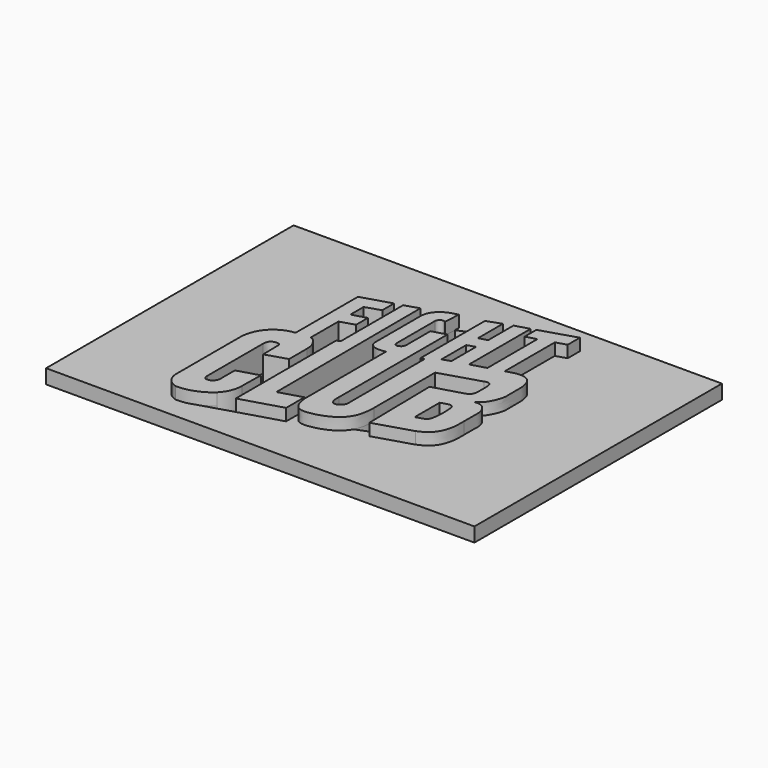
from build123d import *

# Parameters (mm, degrees)
F0_W     = 90
F0_H     = 65
F1_DEPTH = 3
F2_DEPTH = 5.5
F4_DEPTH = 25


# Not quite as in the source:
# - a feature names something its author has since deleted; it is built from what else it names


with BuildPart() as f1:
    # F0 (on Top) → F1 (new body)
    with BuildSketch(Plane.XY):
        Rectangle(F0_W, F0_H)
        with BuildLine():
            Line((-11.7899651246, 17.3868578509), (-11.7899651246, 14.2935177732))
            Line((-11.7899651246, 14.2935177732), (-14.9118620558, 13.28190385))
            Line((-14.9118620558, 13.28190385), (-14.9118620558, 9.8245825553))
            Line((-14.9118620558, 9.8245825553), (-14.8359441439, 9.8464276794))
            Line((-14.8359441439, 9.8464276794), (-11.9289977815, 10.6828917294))
            Line((-11.9289977815, 10.6828917294), (-11.9289977815, 7.5737699435))
            Line((-11.9289977815, 7.5737699435), (-14.9118620558, 6.6583940559))
            Line((-14.9118620558, 6.6583940559), (-14.9118620558, -0.6190531353))
            Line((-14.9118620558, -0.6190531353), (-14.8359441439, -0.6190531353))
            add(Edge.make_bspline(
                [(-12.8983538912, -4.1546191569), (-12.9124355164, -3.4646401315), (-13.0426874661, -2.4052822087), (-14.1635179222, -0.8313651281), (-14.6513370426, -0.6795562339), (-14.8359441439, -0.6190531353)],
                knots=[0, 0, 0, 0, 0.3871210779, 0.7691695686, 1, 1, 1, 1], degree=3))
            Line((-12.8983538912, -4.1546191569), (-12.8983538912, -8.8000393834))
            Line((-12.8983538912, -8.8000393834), (-17.270977576, -10.1718452605))
            Line((-17.270977576, -10.1718452605), (-17.3239837629, -6.5835107489))
            add(Edge.make_bspline(
                [(-19.649932717, -7.1929238033), (-19.6340625481, -6.6727895144), (-19.4415656957, -6.0485860746), (-18.7104823295, -5.5186813522), (-17.3236080712, -5.4227422638), (-17.3243871941, -6.203783376), (-17.3239837629, -6.5835107489)],
                knots=[0, 0, 0, 0, 0.266822824, 0.4960878337, 0.7560668313, 1, 1, 1, 1], degree=3))
            Line((-19.649932717, -7.1929238033), (-19.649932717, -21.7389181386))
            add(Edge.make_bspline(
                [(-18.3777159405, -22.8102611267), (-18.7096900591, -22.8762786233), (-19.33843798, -23.0013135624), (-19.6405821898, -22.1927150073), (-19.6470449505, -21.8790663219), (-19.649932717, -21.7389181386)],
                knots=[0, 0, 0, 0, 0.3822506469, 0.7239699906, 1, 1, 1, 1], degree=3))
            ThreePointArc((-18.3777159405, -22.8102611267), (-17.6136064221, -22.2363913544), (-17.3231101454, -21.3260058399))
            Line((-17.3231101454, -21.3260058399), (-17.3231101454, -17.5101269313))
            Line((-17.3231101454, -17.5101269313), (-12.8908924283, -16.2136158955))
            Line((-12.8908924283, -16.2136158955), (-12.9712542512, -21.1030652423))
            ThreePointArc((-12.9712542512, -21.1030652423), (-13.4353650173, -23.4585093269), (-14.7708491992, -25.4535024695))
            ThreePointArc((-14.7708491992, -25.4535024695), (-17.8496394574, -27.3225084243), (-21.3954732545, -27.9543275408))
            ThreePointArc((-21.3954732545, -27.9543275408), (-23.3162452582, -26.6851378839), (-24.0600023068, -24.5063692115))
            Line((-24.0600023068, -24.5063692115), (-24.0600023068, -8.0969591465))
            ThreePointArc((-24.0600023068, -8.0969591465), (-23.8409881388, -6.008395119), (-23.0513839577, -4.0624783325))
            ThreePointArc((-23.0513839577, -4.0624783325), (-20.856584496, -1.8407427995), (-17.897732893, -0.8415177762))
            Line((-17.897732893, -0.8415177762), (-17.897732893, 15.5245404617))
            Line((-17.897732893, 15.5245404617), (-11.7899651246, 17.3868578509))
        make_face(mode=Mode.SUBTRACT)
        Polygon((-10.2390258983, 17.8220402536), (-7.3459431316, 18.7296739119), (-7.2041264371, -19.249136779), (-2.439048632, -17.8309577456), (-2.439048632, -22.6527638219), (-10.9764799627, -25.2054852029), (-10.9764799627, 1.1442654634), (-10.2390258983, 1.3995376015), align=None, mode=Mode.SUBTRACT)
        with BuildLine():
            add(Edge.make_bspline(
                [(-1.0214279034, 20.9294296394), (-1.795044013, 20.7272698748), (-3.3218007923, 20.3406175558), (-5.1422433593, 18.8024410524), (-5.5532558817, 17.434179196), (-5.6010190581, 16.6460884355)],
                knots=[0, 0, 0, 0, 0.3420427267, 0.6738343467, 1, 1, 1, 1], degree=3))
            Line((-1.0214279034, 20.9294296394), (-1.1788295361, 17.5223806532))
            ThreePointArc((-1.1788295361, 17.5223806532), (-1.3659565648, 17.6186204532), (-1.5723679927, 17.6595221205))
            ThreePointArc((-1.5723679927, 17.6595221205), (-2.3268435709, 17.3860281515), (-2.645024017, 16.6492829086))
            Line((-2.645024017, 16.6492829086), (-2.645024017, 6.6834372087))
            add(Edge.make_bspline(
                [(-0.975842239, 7.3917701397), (-0.9782823928, 7.3091479001), (-0.9566797659, 7.1256039043), (-1.0681286366, 6.5441772072), (-1.3929022467, 6.1116799848), (-2.5109116823, 5.7508045045), (-2.6580041052, 6.412182815), (-2.645024017, 6.6834372087)],
                knots=[0, 0, 0, 0, 0.1336018541, 0.3279707081, 0.5240102199, 0.7751644105, 1, 1, 1, 1], degree=3))
            Line((-0.975842239, 7.3917701397), (-0.975842239, 13.4126014265))
            Line((-0.975842239, 13.4126014265), (1.9419226264, 14.2566961684))
            Line((1.9419226264, 14.2566961684), (1.9419226264, -14.2681037451))
            add(Edge.make_bspline(
                [(4.4582015212, -14.2681037451), (4.4582015212, -14.4613851485), (4.6185530783, -15.2735437801), (3.810378959, -16.3402712665), (2.669439425, -16.7790884746), (1.8680807242, -15.7743077401), (1.9702860752, -14.8211937439), (1.9419226264, -14.2681037451)],
                knots=[0, 0, 0, 0, 0.1782994827, 0.39186138, 0.5816412367, 0.7692567527, 1, 1, 1, 1], degree=3))
            Line((4.4582015212, -14.2681037451), (4.4582015212, 5.1330709979))
            Line((4.4582015212, 5.1330709979), (3.7308113658, 4.9677546006))
            Line((3.7308113658, 4.9677546006), (3.7308113658, 21.8574482525))
            Line((3.7308113658, 21.8574482525), (6.6653340971, 22.8784648276))
            Line((6.6653340971, 22.8784648276), (6.6653340971, 16.368545091))
            Line((6.6653340971, 16.368545091), (8.419302035, 16.8407677776))
            Line((8.419302035, 16.8407677776), (8.419302035, 23.4856081248))
            Line((8.419302035, 23.4856081248), (11.3538244915, 24.3288611169))
            Line((11.3538244915, 24.3288611169), (11.3538244915, 8.1383883934))
            Line((11.3538244915, 8.1383883934), (14.4907289629, 9.0491027897))
            Line((14.4907289629, 9.0491027897), (14.4907289629, 22.1701313472))
            Line((14.4907289629, 22.1701313472), (12.2982687658, 21.56298805))
            Line((12.2982687658, 21.56298805), (12.2982687658, 24.6324316666))
            Line((12.2982687658, 24.6324316666), (19.6177110671, 26.9260831458))
            Line((19.6177110671, 26.9260831458), (19.6177110671, 23.7217178197))
            Line((19.6177110671, 23.7217178197), (17.4389254567, 23.0471158656))
            Line((17.4389254567, 23.0471158656), (17.4389254567, 9.9340454692))
            Line((17.4389254567, 9.9340454692), (17.5568187673, 9.9340454692))
            add(Edge.make_bspline(
                [(23.3318888071, -8.1512481567), (23.3311911227, -7.4858005871), (23.3307677799, -6.4709077438), (23.3343646105, -5.0115116682), (23.3288725027, -4.9910573322), (23.4432301916, -3.9602161044), (22.7653981413, -2.4247467881), (21.4983184593, -1.5549434987), (19.998240636, -1.8718939633), (21.2623812155, -1.1033143641), (22.0502922664, -0.3456082574), (23.2245036891, 2.2173413762), (23.1970215174, 3.8249680988), (23.1643405632, 6.7270889592), (23.1681424876, 7.3536889688), (22.7894330471, 9.4422107912), (21.4631720563, 10.4647739779), (19.6042894167, 10.627637088), (18.2733323534, 10.1767682526), (17.5568187673, 9.9340454692)],
                knots=[0, 0, 0, 0, 0.0686633322, 0.1241792585, 0.1317609375, 0.1781168183, 0.2439866183, 0.3061193494, 0.3529473951, 0.3988783877, 0.455494654, 0.5360218639, 0.6036835088, 0.6857463768, 0.7281580678, 0.797518151, 0.8604110332, 0.9264215245, 1, 1, 1, 1], degree=3))
            add(Edge.make_bspline(
                [(19.2568509865, -15.8505986956), (19.5510345612, -15.7266917741), (20.2459241451, -15.4339755), (21.9033973633, -14.3394960858), (22.9170105079, -12.421003478), (23.3512677684, -10.475815106), (23.3305495269, -8.9474042322), (23.3318888071, -8.1512481567)],
                knots=[0, 0, 0, 0, 0.1499469204, 0.3543171151, 0.5693051427, 0.7758772125, 1, 1, 1, 1], degree=3))
            Line((19.2568509865, -15.8505986956), (11.5152085686, -18.23727121))
            Line((11.5152085686, -18.23727121), (11.2434201144, -2.1050125944))
            Line((11.2434201144, -2.1050125944), (17.0577787685, -0.4173805913))
            add(Edge.make_bspline(
                [(17.0577787685, 4.9326692384), (17.2359444971, 5.0062828452), (17.5963985204, 5.1552133997), (18.3004216541, 5.0379598376), (18.5868743443, 4.0594275645), (18.5659774666, 3.2509662277), (18.6012430245, 1.112721129), (18.3101521273, 0.2135182891), (17.6915830324, -0.2066600599), (17.2685862853, -0.34729354), (17.0577787685, -0.4173805913)],
                knots=[0, 0, 0, 0, 0.1016144921, 0.2055802359, 0.3310055102, 0.4574330561, 0.651788574, 0.7805878019, 0.8906522546, 1, 1, 1, 1], degree=3))
            Line((17.0577787685, 4.9326692384), (8.8136700145, 2.4044824988))
            Line((8.8136700145, 2.4044824988), (8.8136700145, -13.70638746))
            add(Edge.make_bspline(
                [(-2.1296884432, -18.019118476), (-2.0995822923, -18.6635207362), (-1.857078119, -19.823460143), (-1.4816179926, -20.7110735924), (-0.7399237684, -21.5449777161), (0.5509044259, -21.8812292133), (3.1831892549, -21.4471075773), (6.0217835741, -20.2553038527), (7.6687373415, -18.601967223), (8.4960625988, -16.8878330756), (8.8140079, -14.7485973532), (8.8137678216, -14.0086200559), (8.8136700145, -13.70638746)],
                knots=[0, 0, 0, 0, 0.1027277517, 0.1769473417, 0.2532577584, 0.3376408889, 0.4609102569, 0.5950787177, 0.7085765562, 0.813280218, 0.9237370973, 1, 1, 1, 1], degree=3))
            Line((-2.1296884432, -18.019118476), (-2.1296884432, 3.1618176804))
            Line((-2.1296884432, 3.1618176804), (-2.2223336581, 3.1618176804))
            add(Edge.make_bspline(
                [(-5.6010190581, 4.5141229309), (-5.5493043432, 3.954976001), (-4.844515491, 3.1292890206), (-3.2977966838, 2.9514441965), (-2.5561304606, 3.0983845963), (-2.2223336581, 3.1618176804)],
                knots=[0, 0, 0, 0, 0.3499782987, 0.7004813403, 1, 1, 1, 1], degree=3))
            Line((-5.6010190581, 4.5141229309), (-5.6010190581, 16.6460884355))
        make_face(mode=Mode.SUBTRACT)
    extrude(amount=F1_DEPTH)

    # F0 (on Top) → F2 (join)
    with BuildSketch(Plane.XY):
        with BuildLine():
            Line((-14.9118620558, 13.28190385), (-11.7899651246, 14.2935177732))
            Line((-11.7899651246, 14.2935177732), (-11.7899651246, 17.3868578509))
            Line((-11.7899651246, 17.3868578509), (-17.897732893, 15.5245404617))
            Line((-17.897732893, 15.5245404617), (-17.897732893, -0.8415177762))
            ThreePointArc((-17.897732893, -0.8415177762), (-20.856584496, -1.8407427995), (-23.0513839577, -4.0624783325))
            ThreePointArc((-23.0513839577, -4.0624783325), (-23.8409881388, -6.008395119), (-24.0600023068, -8.0969591465))
            Line((-24.0600023068, -8.0969591465), (-24.0600023068, -24.5063692115))
            ThreePointArc((-24.0600023068, -24.5063692115), (-23.3162452582, -26.6851378839), (-21.3954732545, -27.9543275408))
            ThreePointArc((-21.3954732545, -27.9543275408), (-17.8496394574, -27.3225084243), (-14.7708491992, -25.4535024695))
            ThreePointArc((-14.7708491992, -25.4535024695), (-13.4353650173, -23.4585093269), (-12.9712542512, -21.1030652423))
            Line((-12.9712542512, -21.1030652423), (-12.8908924283, -16.2136158955))
            Line((-12.8908924283, -16.2136158955), (-17.3231101454, -17.5101269313))
            Line((-17.3231101454, -17.5101269313), (-17.3231101454, -21.3260058399))
            ThreePointArc((-17.3231101454, -21.3260058399), (-17.6136064221, -22.2363913544), (-18.3777159405, -22.8102611267))
            add(Edge.make_bspline(
                [(-18.3777159405, -22.8102611267), (-18.7096900591, -22.8762786233), (-19.33843798, -23.0013135624), (-19.6405821898, -22.1927150073), (-19.6470449505, -21.8790663219), (-19.649932717, -21.7389181386)],
                knots=[0, 0, 0, 0, 0.3822506469, 0.7239699906, 1, 1, 1, 1], degree=3))
            Line((-19.649932717, -21.7389181386), (-19.649932717, -7.1929238033))
            add(Edge.make_bspline(
                [(-19.649932717, -7.1929238033), (-19.6340625481, -6.6727895144), (-19.4415656957, -6.0485860746), (-18.7104823295, -5.5186813522), (-17.3236080712, -5.4227422638), (-17.3243871941, -6.203783376), (-17.3239837629, -6.5835107489)],
                knots=[0, 0, 0, 0, 0.266822824, 0.4960878337, 0.7560668313, 1, 1, 1, 1], degree=3))
            Line((-17.3239837629, -6.5835107489), (-17.270977576, -10.1718452605))
            Line((-17.270977576, -10.1718452605), (-12.8983538912, -8.8000393834))
            Line((-12.8983538912, -8.8000393834), (-12.8983538912, -4.1546191569))
            add(Edge.make_bspline(
                [(-12.8983538912, -4.1546191569), (-12.9124355164, -3.4646401315), (-13.0426874661, -2.4052822087), (-14.1635179222, -0.8313651281), (-14.6513370426, -0.6795562339), (-14.8359441439, -0.6190531353)],
                knots=[0, 0, 0, 0, 0.3871210779, 0.7691695686, 1, 1, 1, 1], degree=3))
            Line((-14.8359441439, -0.6190531353), (-14.9118620558, -0.6190531353))
            Line((-14.9118620558, -0.6190531353), (-14.9118620558, 6.6583940559))
            Line((-14.9118620558, 6.6583940559), (-11.9289977815, 7.5737699435))
            Line((-11.9289977815, 7.5737699435), (-11.9289977815, 10.6828917294))
            Line((-11.9289977815, 10.6828917294), (-14.8359441439, 9.8464276794))
            Line((-14.8359441439, 9.8464276794), (-14.9118620558, 9.8245825553))
            Line((-14.9118620558, 9.8245825553), (-14.9118620558, 13.28190385))
        make_face()
        Polygon((-7.2041264371, -19.249136779), (-7.3459431316, 18.7296739119), (-10.2390258983, 17.8220402536), (-10.2390258983, 1.3995376015), (-10.9764799627, 1.1442654634), (-10.9764799627, -25.2054852029), (-2.439048632, -22.6527638219), (-2.439048632, -17.8309577456), align=None)
        with BuildLine():
            Line((-1.1788295361, 17.5223806532), (-1.0214279034, 20.9294296394))
            add(Edge.make_bspline(
                [(-1.0214279034, 20.9294296394), (-1.795044013, 20.7272698748), (-3.3218007923, 20.3406175558), (-5.1422433593, 18.8024410524), (-5.5532558817, 17.434179196), (-5.6010190581, 16.6460884355)],
                knots=[0, 0, 0, 0, 0.3420427267, 0.6738343467, 1, 1, 1, 1], degree=3))
            Line((-5.6010190581, 16.6460884355), (-5.6010190581, 4.5141229309))
            add(Edge.make_bspline(
                [(-5.6010190581, 4.5141229309), (-5.5493043432, 3.954976001), (-4.844515491, 3.1292890206), (-3.2977966838, 2.9514441965), (-2.5561304606, 3.0983845963), (-2.2223336581, 3.1618176804)],
                knots=[0, 0, 0, 0, 0.3499782987, 0.7004813403, 1, 1, 1, 1], degree=3))
            Line((-2.2223336581, 3.1618176804), (-2.1296884432, 3.1618176804))
            Line((-2.1296884432, 3.1618176804), (-2.1296884432, -18.019118476))
            add(Edge.make_bspline(
                [(-2.1296884432, -18.019118476), (-2.0995822923, -18.6635207362), (-1.857078119, -19.823460143), (-1.4816179926, -20.7110735924), (-0.7399237684, -21.5449777161), (0.5509044259, -21.8812292133), (3.1831892549, -21.4471075773), (6.0217835741, -20.2553038527), (7.6687373415, -18.601967223), (8.4960625988, -16.8878330756), (8.8140079, -14.7485973532), (8.8137678216, -14.0086200559), (8.8136700145, -13.70638746)],
                knots=[0, 0, 0, 0, 0.1027277517, 0.1769473417, 0.2532577584, 0.3376408889, 0.4609102569, 0.5950787177, 0.7085765562, 0.813280218, 0.9237370973, 1, 1, 1, 1], degree=3))
            Line((8.8136700145, -13.70638746), (8.8136700145, 2.4044824988))
            Line((8.8136700145, 2.4044824988), (17.0577787685, 4.9326692384))
            add(Edge.make_bspline(
                [(17.0577787685, 4.9326692384), (17.2359444971, 5.0062828452), (17.5963985204, 5.1552133997), (18.3004216541, 5.0379598376), (18.5868743443, 4.0594275645), (18.5659774666, 3.2509662277), (18.6012430245, 1.112721129), (18.3101521273, 0.2135182891), (17.6915830324, -0.2066600599), (17.2685862853, -0.34729354), (17.0577787685, -0.4173805913)],
                knots=[0, 0, 0, 0, 0.1016144921, 0.2055802359, 0.3310055102, 0.4574330561, 0.651788574, 0.7805878019, 0.8906522546, 1, 1, 1, 1], degree=3))
            Line((17.0577787685, -0.4173805913), (11.2434201144, -2.1050125944))
            Line((11.2434201144, -2.1050125944), (11.5152085686, -18.23727121))
            Line((11.5152085686, -18.23727121), (19.2568509865, -15.8505986956))
            add(Edge.make_bspline(
                [(19.2568509865, -15.8505986956), (19.5510345612, -15.7266917741), (20.2459241451, -15.4339755), (21.9033973633, -14.3394960858), (22.9170105079, -12.421003478), (23.3512677684, -10.475815106), (23.3305495269, -8.9474042322), (23.3318888071, -8.1512481567)],
                knots=[0, 0, 0, 0, 0.1499469204, 0.3543171151, 0.5693051427, 0.7758772125, 1, 1, 1, 1], degree=3))
            add(Edge.make_bspline(
                [(23.3318888071, -8.1512481567), (23.3311911227, -7.4858005871), (23.3307677799, -6.4709077438), (23.3343646105, -5.0115116682), (23.3288725027, -4.9910573322), (23.4432301916, -3.9602161044), (22.7653981413, -2.4247467881), (21.4983184593, -1.5549434987), (19.998240636, -1.8718939633), (21.2623812155, -1.1033143641), (22.0502922664, -0.3456082574), (23.2245036891, 2.2173413762), (23.1970215174, 3.8249680988), (23.1643405632, 6.7270889592), (23.1681424876, 7.3536889688), (22.7894330471, 9.4422107912), (21.4631720563, 10.4647739779), (19.6042894167, 10.627637088), (18.2733323534, 10.1767682526), (17.5568187673, 9.9340454692)],
                knots=[0, 0, 0, 0, 0.0686633322, 0.1241792585, 0.1317609375, 0.1781168183, 0.2439866183, 0.3061193494, 0.3529473951, 0.3988783877, 0.455494654, 0.5360218639, 0.6036835088, 0.6857463768, 0.7281580678, 0.797518151, 0.8604110332, 0.9264215245, 1, 1, 1, 1], degree=3))
            Line((17.5568187673, 9.9340454692), (17.4389254567, 9.9340454692))
            Line((17.4389254567, 9.9340454692), (17.4389254567, 23.0471158656))
            Line((17.4389254567, 23.0471158656), (19.6177110671, 23.7217178197))
            Line((19.6177110671, 23.7217178197), (19.6177110671, 26.9260831458))
            Line((19.6177110671, 26.9260831458), (12.2982687658, 24.6324316666))
            Line((12.2982687658, 24.6324316666), (12.2982687658, 21.56298805))
            Line((12.2982687658, 21.56298805), (14.4907289629, 22.1701313472))
            Line((14.4907289629, 22.1701313472), (14.4907289629, 9.0491027897))
            Line((14.4907289629, 9.0491027897), (11.3538244915, 8.1383883934))
            Line((11.3538244915, 8.1383883934), (11.3538244915, 24.3288611169))
            Line((11.3538244915, 24.3288611169), (8.419302035, 23.4856081248))
            Line((8.419302035, 23.4856081248), (8.419302035, 16.8407677776))
            Line((8.419302035, 16.8407677776), (6.6653340971, 16.368545091))
            Line((6.6653340971, 16.368545091), (6.6653340971, 22.8784648276))
            Line((6.6653340971, 22.8784648276), (3.7308113658, 21.8574482525))
            Line((3.7308113658, 21.8574482525), (3.7308113658, 4.9677546006))
            Line((3.7308113658, 4.9677546006), (4.4582015212, 5.1330709979))
            Line((4.4582015212, 5.1330709979), (4.4582015212, -14.2681037451))
            add(Edge.make_bspline(
                [(4.4582015212, -14.2681037451), (4.4582015212, -14.4613851485), (4.6185530783, -15.2735437801), (3.810378959, -16.3402712665), (2.669439425, -16.7790884746), (1.8680807242, -15.7743077401), (1.9702860752, -14.8211937439), (1.9419226264, -14.2681037451)],
                knots=[0, 0, 0, 0, 0.1782994827, 0.39186138, 0.5816412367, 0.7692567527, 1, 1, 1, 1], degree=3))
            Line((1.9419226264, -14.2681037451), (1.9419226264, 14.2566961684))
            Line((1.9419226264, 14.2566961684), (-0.975842239, 13.4126014265))
            Line((-0.975842239, 13.4126014265), (-0.975842239, 7.3917701397))
            add(Edge.make_bspline(
                [(-0.975842239, 7.3917701397), (-0.9782823928, 7.3091479001), (-0.9566797659, 7.1256039043), (-1.0681286366, 6.5441772072), (-1.3929022467, 6.1116799848), (-2.5109116823, 5.7508045045), (-2.6580041052, 6.412182815), (-2.645024017, 6.6834372087)],
                knots=[0, 0, 0, 0, 0.1336018541, 0.3279707081, 0.5240102199, 0.7751644105, 1, 1, 1, 1], degree=3))
            Line((-2.645024017, 6.6834372087), (-2.645024017, 16.6492829086))
            ThreePointArc((-2.645024017, 16.6492829086), (-2.3268435709, 17.3860281515), (-1.5723679927, 17.6595221205))
            ThreePointArc((-1.5723679927, 17.6595221205), (-1.3659565648, 17.6186204532), (-1.1788295361, 17.5223806532))
        make_face()
        with BuildLine():
            Line((16.0750909258, -12.0350967062), (16.0750909258, -5.4968190153))
            add(Edge.make_bspline(
                [(17.6795768623, -11.5336951944), (17.8920563941, -11.4262280449), (18.3973710248, -11.1706517899), (18.7372988579, -9.7112596405), (18.8376836014, -7.3755139415), (18.6614634799, -5.1640350789), (17.8241244526, -4.8737211622), (16.7521460752, -5.2556163147), (16.0750909258, -5.4968190153)],
                knots=[0, 0, 0, 0, 0.117623989, 0.2797310501, 0.5013811183, 0.6992003261, 0.8100167201, 1, 1, 1, 1], degree=3))
            Line((17.6795768623, -11.5336951944), (16.0750909258, -12.0350967062))
        make_face(mode=Mode.SUBTRACT)
        Polygon((6.6888508901, 6.7173264257), (6.6888508901, 13.2154924352), (8.3535043486, 13.7369497876), (8.3535043486, 7.2588401683), align=None, mode=Mode.SUBTRACT)
    extrude(amount=F2_DEPTH)

    # F3 (on face) → F4 (cut)
    with BuildSketch(Plane.XY.offset(3)):
        with BuildLine():
            ThreePointArc((-14.7708491992, -25.4535024695), (-16.1157857913, -26.464031922), (-17.6136064221, -27.2299023868))
            Line((-17.6136064221, -27.2299023868), (-10.9764799627, -25.2054852029))
            Line((-10.9764799627, -25.2054852029), (-10.9764799627, 1.1442654634))
            Line((-10.9764799627, 1.1442654634), (-10.2390258983, 1.3995376015))
            Line((-10.2390258983, 1.3995376015), (-10.2390258983, 17.8220402536))
            Line((-10.2390258983, 17.8220402536), (-7.3459431316, 18.7296739119))
            Line((-7.3459431316, 18.7296739119), (-11.7899651246, 17.3868578509))
            Line((-11.7899651246, 17.3868578509), (-11.7899651246, 14.2935177732))
            Line((-11.7899651246, 14.2935177732), (-14.9118620558, 13.28190385))
            Line((-14.9118620558, 13.28190385), (-14.9118620558, 9.8245825553))
            Line((-14.9118620558, 9.8245825553), (-11.9289977815, 10.6828917294))
            Line((-11.9289977815, 10.6828917294), (-11.9289977815, 7.5737699435))
            Line((-11.9289977815, 7.5737699435), (-14.9118620558, 6.6583940559))
            Line((-14.9118620558, 6.6583940559), (-14.9118620558, -0.6190531353))
            Line((-14.9118620558, -0.6190531353), (-14.8359441439, -0.6190531353))
            add(Edge.make_bspline(
                [(-12.8983538912, -4.1546191569), (-12.9124355164, -3.4646401315), (-13.0426874661, -2.4052822087), (-14.1635179222, -0.8313651281), (-14.6513370426, -0.6795562339), (-14.8359441439, -0.6190531353)],
                knots=[0, 0, 0, 0, 0.3871210779, 0.7691695686, 1, 1, 1, 1], degree=3))
            Line((-12.8983538912, -4.1546191569), (-12.8983538912, -8.8000393834))
            Line((-12.8983538912, -8.8000393834), (-17.270977576, -10.1718452605))
            Line((-17.270977576, -10.1718452605), (-17.3239837629, -6.5835107489))
            add(Edge.make_bspline(
                [(-19.649932717, -7.1929238033), (-19.6340625481, -6.6727895144), (-19.4415656957, -6.0485860746), (-18.7104823295, -5.5186813522), (-17.3236080712, -5.4227422638), (-17.3243871941, -6.203783376), (-17.3239837629, -6.5835107489)],
                knots=[0, 0, 0, 0, 0.266822824, 0.4960878337, 0.7560668313, 1, 1, 1, 1], degree=3))
            Line((-19.649932717, -7.1929238033), (-19.649932717, -21.7389181386))
            add(Edge.make_bspline(
                [(-18.3777159405, -22.8102611267), (-18.7096900591, -22.8762786233), (-19.33843798, -23.0013135624), (-19.6405821898, -22.1927150073), (-19.6470449505, -21.8790663219), (-19.649932717, -21.7389181386)],
                knots=[0, 0, 0, 0, 0.3822506469, 0.7239699906, 1, 1, 1, 1], degree=3))
            ThreePointArc((-18.3777159405, -22.8102611267), (-17.6136064221, -22.2363913544), (-17.3231101454, -21.3260058399))
            Line((-17.3231101454, -21.3260058399), (-17.3231101454, -17.5101269313))
            Line((-17.3231101454, -17.5101269313), (-12.8908924283, -16.2136158955))
            Line((-12.8908924283, -16.2136158955), (-12.9712542512, -21.1030652423))
            ThreePointArc((-12.9712542512, -21.1030652423), (-13.4353650173, -23.4585093269), (-14.7708491992, -25.4535024695))
        make_face()
        Polygon((12.2982687658, 24.6324316666), (11.3538244915, 24.3288611169), (11.3538244915, 8.1383883934), (14.4907289629, 9.0491027897), (14.4907289629, 22.1701313472), (12.2982687658, 21.56298805), align=None)
        Polygon((8.419302035, 23.4856081248), (6.6653340971, 22.8784648276), (6.6653340971, 16.368545091), (8.419302035, 16.8407677776), align=None)
        with BuildLine():
            Line((-7.2041264371, -19.249136779), (-2.439048632, -17.8309577456))
            Line((-2.439048632, -17.8309577456), (-2.1296884432, -17.8309577456))
            Line((-2.1296884432, -17.8309577456), (-2.1296884432, 3.1618176804))
            Line((-2.1296884432, 3.1618176804), (-2.2223336581, 3.1618176804))
            add(Edge.make_bspline(
                [(-5.6010190581, 4.5141229309), (-5.5493043432, 3.954976001), (-4.844515491, 3.1292890206), (-3.2977966838, 2.9514441965), (-2.5561304606, 3.0983845963), (-2.2223336581, 3.1618176804)],
                knots=[0, 0, 0, 0, 0.3499782987, 0.7004813403, 1, 1, 1, 1], degree=3))
            Line((-5.6010190581, 4.5141229309), (-5.6010190581, 16.6460884355))
            add(Edge.make_bspline(
                [(-4.5502084243, 19.2051618362), (-4.6992452205, 19.0466929058), (-5.288938287, 18.3140932208), (-5.5532558817, 17.434179196), (-5.6010190581, 16.6460884355)],
                knots=[0.5768749748, 0.5768749748, 0.5768749748, 0.5768749748, 0.6738343467, 1, 1, 1, 1], degree=3))
            Line((-4.5502084243, 19.2051618362), (-7.3451423339, 18.5152185953))
            Line((-7.3451423339, 18.5152185953), (-7.2041264371, -19.249136779))
        make_face()
        with BuildLine():
            Line((3.7308113658, 21.8574482525), (-1.065978984, 19.9650958431))
            Line((-1.065978984, 19.9650958431), (-1.1788295361, 17.5223806532))
            ThreePointArc((-1.1788295361, 17.5223806532), (-1.3659565648, 17.6186204532), (-1.5723679927, 17.6595221205))
            ThreePointArc((-1.5723679927, 17.6595221205), (-2.3268435709, 17.3860281515), (-2.645024017, 16.6492829086))
            Line((-2.645024017, 16.6492829086), (-2.645024017, 6.6834372087))
            add(Edge.make_bspline(
                [(-0.975842239, 7.3917701397), (-0.9782823928, 7.3091479001), (-0.9566797659, 7.1256039043), (-1.0681286366, 6.5441772072), (-1.3929022467, 6.1116799848), (-2.5109116823, 5.7508045045), (-2.6580041052, 6.412182815), (-2.645024017, 6.6834372087)],
                knots=[0, 0, 0, 0, 0.1336018541, 0.3279707081, 0.5240102199, 0.7751644105, 1, 1, 1, 1], degree=3))
            Line((-0.975842239, 7.3917701397), (-0.975842239, 13.4126014265))
            Line((-0.975842239, 13.4126014265), (1.9419226264, 14.2566961684))
            Line((1.9419226264, 14.2566961684), (1.9419226264, -14.2681037451))
            add(Edge.make_bspline(
                [(4.4582015212, -14.2681037451), (4.4582015212, -14.4613851485), (4.6185530783, -15.2735437801), (3.810378959, -16.3402712665), (2.669439425, -16.7790884746), (1.8680807242, -15.7743077401), (1.9702860752, -14.8211937439), (1.9419226264, -14.2681037451)],
                knots=[0, 0, 0, 0, 0.1782994827, 0.39186138, 0.5816412367, 0.7692567527, 1, 1, 1, 1], degree=3))
            Line((4.4582015212, -14.2681037451), (4.4582015212, 5.1330709979))
            Line((4.4582015212, 5.1330709979), (3.7308113658, 4.9677546006))
            Line((3.7308113658, 4.9677546006), (3.7308113658, 21.8574482525))
        make_face()
        with BuildLine():
            add(Edge.make_bspline(
                [(7.9517668122, -17.9395415215), (8.1390595648, -17.5922634094), (8.538213881, -16.604226027), (8.8140079, -14.7485973532), (8.8137678216, -14.0086200559), (8.8136700145, -13.70638746)],
                knots=[0.7472117294, 0.7472117294, 0.7472117294, 0.7472117294, 0.813280218, 0.9237370973, 1, 1, 1, 1], degree=3))
            Line((7.9517668122, -17.9395415215), (11.4873149812, -16.5816211659))
            Line((11.4873149812, -16.5816211659), (11.2434201144, -2.1050125944))
            Line((11.2434201144, -2.1050125944), (17.0577787685, -0.4173805913))
            add(Edge.make_bspline(
                [(17.0577787685, 4.9326692384), (17.2359444971, 5.0062828452), (17.5963985204, 5.1552133997), (18.3004216541, 5.0379598376), (18.5868743443, 4.0594275645), (18.5659774666, 3.2509662277), (18.6012430245, 1.112721129), (18.3101521273, 0.2135182891), (17.6915830324, -0.2066600599), (17.2685862853, -0.34729354), (17.0577787685, -0.4173805913)],
                knots=[0, 0, 0, 0, 0.1016144921, 0.2055802359, 0.3310055102, 0.4574330561, 0.651788574, 0.7805878019, 0.8906522546, 1, 1, 1, 1], degree=3))
            Line((17.0577787685, 4.9326692384), (8.8136700145, 2.4044824988))
            Line((8.8136700145, 2.4044824988), (8.8136700145, -13.70638746))
        make_face()
    extrude(amount=-F4_DEPTH, mode=Mode.SUBTRACT)


solid = f1.part
